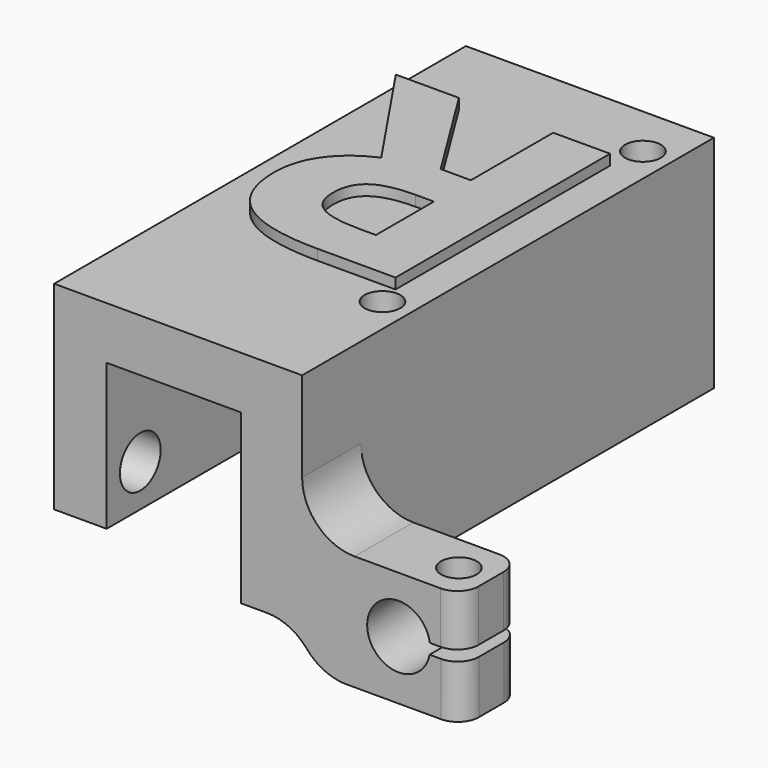
from build123d import *

# Parameters (mm, degrees)
F1_DEPTH      = 7
F2_DEPTH      = 42
F3_R          = 1.7
F3_R_2        = 11
F4_DEPTH      = 21.001
F5_R          = 3
F6_DEPTH      = 10
F7_DEPTH      = 21.001
F8_R          = 1.4
F9_DEPTH      = 11.0176173191
F8_R_2        = 1.7
F10_DEPTH     = 4.9085948419
F11_R         = 5
F12_R         = 5
F13_R         = 5
F14_R         = 2
F15_R         = 2.2
F15_R_2       = 2.4255023423
F16_DEPTH     = 6
F17_TEXT_SIZE = 35.7644961357
F18_DEPTH     = 1


# Not quite as in the source:
# - a feature names something its author has since deleted; it is built from what else it names
# - Text() gives the source's letters only with a copy of the font that has no kerning and outlines rounded to 1/6400 em; it was checked with that copy


with BuildPart() as f1:
    # F0 (on Front) → F1 (new body)
    with BuildSketch(Plane.XZ):
        Polygon((-18.6721007523, 29.8099789735), (-18.6721007523, 10.8925135386), (-13.6721007523, 10.8925135386), (-13.6721007523, 24.8099789735), (-0.8721007523, 24.8099789735), (-0.8721007523, 8.8099789735), (4.9380548998, 8.8099789735), (4.9380548998, 16.2656020473), (4.9380548998, 29.8099789735), align=None)
        Polygon((20.1263195603, 16.2417280634), (4.9380548998, 16.2656020473), (4.9380548998, 8.8099789735), (6.3533044869, 5.2860832236), (20.1553367778, 5.2860832236), (20.1553367778, 10.343908232), (13.4860510706, 10.343908232), (13.4860510706, 11.3388913612), (20.1263195603, 11.3388913612), align=None)
    extrude(amount=F1_DEPTH)

    # F0 (on Front) → F2 (join)
    with BuildSketch(Plane.XZ):
        Polygon((-18.6721007523, 29.8099789735), (-18.6721007523, 10.8925135386), (-13.6721007523, 10.8925135386), (-13.6721007523, 24.8099789735), (-0.8721007523, 24.8099789735), (-0.8721007523, 8.8099789735), (4.9380548998, 8.8099789735), (4.9380548998, 16.2656020473), (4.9380548998, 29.8099789735), align=None)
    extrude(amount=-F2_DEPTH)

    # F3 (on face) → F4 (cut, through all)
    with BuildSketch(Plane(origin=(0, 0, 8.8099789735), x_dir=(1, 0, 0), z_dir=(0, 0, -1))):
        with Locations((2.1850741468, -6)):
            Circle(F3_R)
        with Locations((2.1850741468, -37)):
            Circle(F3_R)
        with Locations((17.6850741468, -21.5)):
            Circle(F3_R_2)
    extrude(amount=-F4_DEPTH, mode=Mode.SUBTRACT)

    # F5 (on face) → F6 (cut)
    with BuildSketch(Plane.XZ.offset(7)):
        with Locations((14.1278992477, 10.8989789735)):
            Circle(F5_R)
    extrude(amount=-F6_DEPTH, mode=Mode.SUBTRACT)

    # F3 (on face) → F7 (cut, through all)
    with BuildSketch(Plane(origin=(0, 0, 8.8099789735), x_dir=(1, 0, 0), z_dir=(0, 0, -1))):
        with Locations((2.1850741468, -6)):
            Circle(F3_R)
        with Locations((2.1850741468, -37)):
            Circle(F3_R)
        with Locations((17.6850741468, -21.5)):
            Circle(F3_R_2)
    extrude(amount=-F7_DEPTH, mode=Mode.SUBTRACT)

    # F8 (on face) → F9 (cut, through all)
    with BuildSketch(Plane(origin=(0.0255795563, 0, 16.273323822), x_dir=(0.9999987646, 0, -0.0015718685), z_dir=(0.0015718685, 0, 0.9999987646))):
        with Locations((17.1007648362, -3.5767070949)):
            Circle(F8_R)
    extrude(amount=-F9_DEPTH, mode=Mode.SUBTRACT)

    # F8 (on face) → F10 (cut, through all)
    with BuildSketch(Plane(origin=(0.0255795563, 0, 16.273323822), x_dir=(0.9999987646, 0, -0.0015718685), z_dir=(0.0015718685, 0, 0.9999987646))):
        with Locations((17.1007648362, -3.5767070949)):
            Circle(F8_R_2)
        with Locations((17.1007648362, -3.5767070949)):
            Circle(F8_R, mode=Mode.SUBTRACT)
    extrude(amount=-F10_DEPTH, mode=Mode.SUBTRACT)

    # F11
    f11_edges = [f1.edges().sort_by_distance(p)[0] for p in [
        (4.938055, -3.5, 16.265602),
    ]]
    fillet(f11_edges, radius=F11_R)

    # F12
    f12_edges = [f1.edges().sort_by_distance(p)[0] for p in [
        (4.938055, -3.5, 8.809979),
    ]]
    fillet(f12_edges, radius=F12_R)

    # F13
    f13_edges = [f1.edges().sort_by_distance(p)[0] for p in [
        (6.353304, -3.5, 5.286083),
    ]]
    fillet(f13_edges, radius=F13_R)

    # F14
    f14_edges = [f1.edges().sort_by_distance(p)[0] for p in [
        (20.12632, -7, 13.79031),
        (20.155337, -7, 7.814996),
        (20.12632, 0, 13.79031),
        (20.155337, 0, 7.814996),
    ]]
    fillet(f14_edges, radius=F14_R)

    # F15 (on face) → F16 (cut)
    with BuildSketch(Plane(origin=(-18.6721007523, 0, 0), x_dir=(0, -1, 0), z_dir=(-1, 0, 0))):
        with Locations((-38, 14.8925135386)):
            Circle(F15_R)
        with Locations((3, 14.8925135386)):
            Circle(F15_R_2)
    extrude(amount=-F16_DEPTH, mode=Mode.SUBTRACT)

    # F17 (on face) → F18 (join)
    with BuildSketch(Plane.XY.offset(29.8099789735)):
        with Locations(Location((4.9380548998, 33.6637421799), (0, 0, 180))):
            Text('R', F17_TEXT_SIZE, font='Open Sans', font_style=FontStyle.BOLD, text_align=(TextAlign.LEFT, TextAlign.BOTTOM))
    extrude(amount=F18_DEPTH)


solid = f1.part
